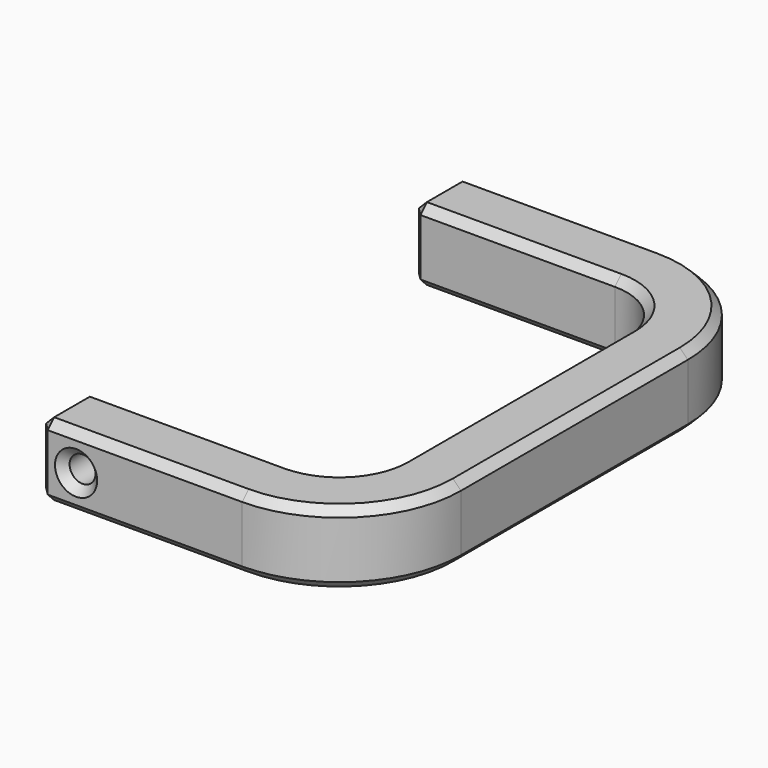
from build123d import *

# Parameters (mm, degrees)
F0_W     = 9
F0_H     = 15
F0_W_2   = 3.2
F1_DEPTH = 9
F3_SIZE  = 2


# Not quite as in the source:
# - a feature names something its author has since deleted; it is built from what else it names


with BuildPart() as f1:
    # F0 (on Top) → F1 (new body, symmetric)
    with BuildSketch(Plane.XY):
        with Locations((-4.5, -7.5)):
            Rectangle(F0_W, F0_H)
        with Locations((1.6, -7.5)):
            Rectangle(F0_W_2, F0_H)
        with BuildLine():
            Line((41, 0), (3.2, 0))
            Line((3.2, 0), (3.2, -15))
            Line((3.2, -15), (41, -15))
            ThreePointArc((41, -15), (62.2132034356, -6.2132034356), (71, 15))
            Line((71, 15), (71, 85))
            ThreePointArc((71, 85), (62.2132034356, 106.2132034356), (41, 115))
            Line((41, 115), (-9, 115))
            Line((-9, 115), (-9, 100))
            Line((-9, 100), (41, 100))
            ThreePointArc((41, 100), (51.6066017178, 95.6066017178), (56, 85))
            Line((56, 85), (56, 15))
            ThreePointArc((56, 15), (51.6066017178, 4.3933982822), (41, 0))
        make_face()
    extrude(amount=F1_DEPTH, both=True)

    # F0 (on Top) → F2 (revolve, cut)
    with BuildSketch(Plane.XY):
        with Locations((1.6, -7.5)):
            Rectangle(F0_W_2, F0_H)
    revolve(axis=Axis((0, -7.5, 0), (0, -1, 0)), mode=Mode.SUBTRACT)

    # F3
    f3_edges = [f1.edges().sort_by_distance(p)[0] for p in [
        (-9, -7.5, 9),
        (16, -15, 9),
        (62.213203, -6.213203, 9),
        (71, 50, 9),
        (62.213203, 106.213203, 9),
        (16, 115, 9),
        (-9, 107.5, 9),
        (16, 100, 9),
        (51.606602, 95.606602, 9),
        (56, 50, 9),
        (51.606602, 4.393398, 9),
        (16, 0, 9),
        (-9, -7.5, -9),
        (16, -15, -9),
        (62.213203, -6.213203, -9),
        (71, 50, -9),
        (62.213203, 106.213203, -9),
        (16, 115, -9),
        (-9, 107.5, -9),
        (16, 100, -9),
        (51.606602, 95.606602, -9),
        (56, 50, -9),
        (51.606602, 4.393398, -9),
        (16, 0, -9),
        (-9, -15, 0),
        (-9, 0, 0),
        (-9, 115, 0),
        (-9, 100, 0),
        (-3.2, -15, 0),
        (-3.2, 0, 0),
    ]]
    chamfer(f3_edges, length=F3_SIZE)


solid = f1.part
